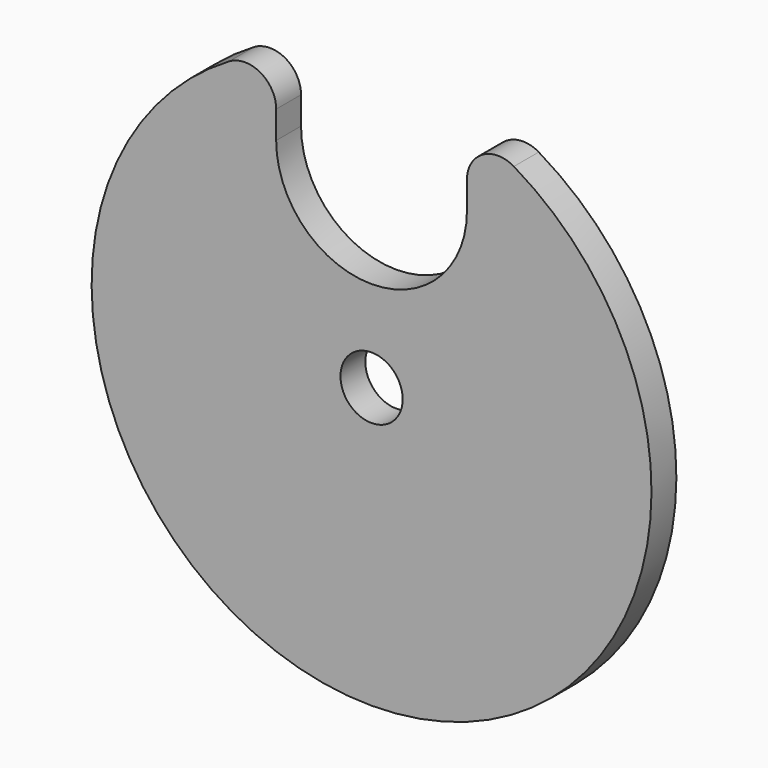
from build123d import *

# Parameters (mm, degrees)
F0_R     = 27
F0_R_2   = 3
F1_DEPTH = 3
F3_DEPTH = 3
F4_R     = 3


# Not quite as in the source:
# - a feature names something its author has since deleted; it is built from what else it names


with BuildPart() as f1:
    # F0 (on Front) → F1 (new body)
    with BuildSketch(Plane.XZ):
        Circle(F0_R)
        Circle(F0_R_2, mode=Mode.SUBTRACT)
    extrude(amount=F1_DEPTH)

    # F2 (on face) → F3 (cut)
    with BuildSketch(Plane.XZ.offset(3)):
        with BuildLine():
            Line((-9.2, 30.5910954097), (-9.2, 18))
            ThreePointArc((-9.2, 18), (0, 8.8), (9.2, 18))
            Line((9.2, 18), (9.2, 30.5910954097))
            Line((9.2, 30.5910954097), (-9.2, 30.5910954097))
        make_face()
    extrude(amount=-F3_DEPTH, mode=Mode.SUBTRACT)

    # F4
    f4_edges = [f1.edges().sort_by_distance(p)[0] for p in [
        (-9.2, -1.5, 25.384247),
        (9.2, -1.5, 25.384247),
    ]]
    fillet(f4_edges, radius=F4_R)


solid = f1.part
